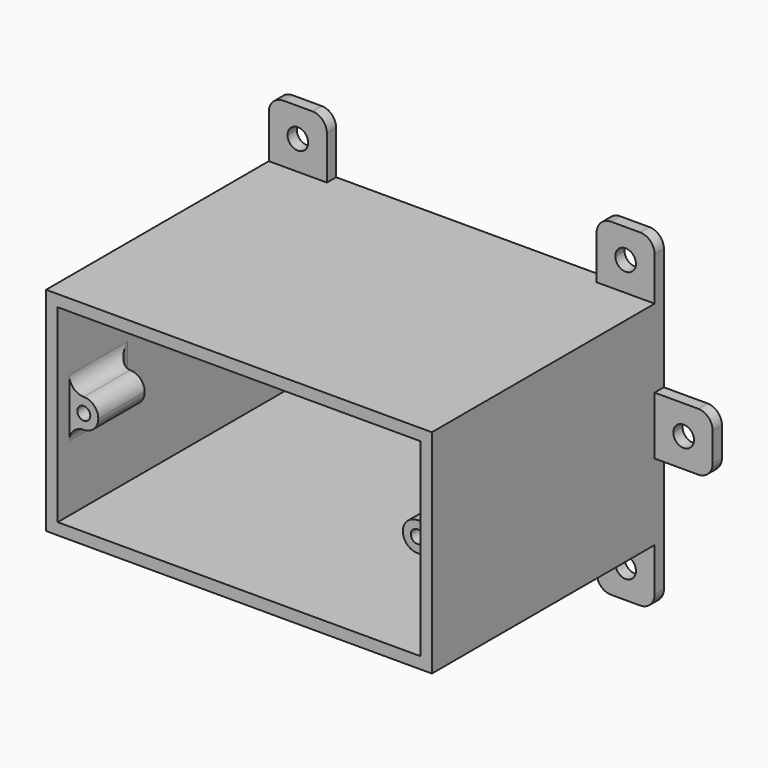
from build123d import *

# Parameters (mm, degrees)
F1_DEPTH     = 40
F0_W         = 8
F0_H         = 8
F0_R         = 1.425
F2_DEPTH     = 1.6
F3_R         = 2
F5_R         = 2
F6_START     = 30
F0_W_2       = 4
F0_H_2       = 4
F0_R_2       = 0.9
F6_DEPTH     = 8
F7_T1_DEPTH  = 8
F7_T6_DEPTH  = 4
F7_S7_R      = 0.9
F7_T8_DEPTH  = 4
F7_T13_DEPTH = 9
F7_T17_DEPTH = 13
F7_T24_DEPTH = 9
F7_T28_DEPTH = 13
F7_T31_DEPTH = 18


# Not quite as in the source:
# - a fillet or chamfer that OpenCascade refuses, or shapes differently, is made with other operations: its cross-section is extruded or revolved along the edge and cut away or added


with BuildPart() as f1:
    # F0 (on Front) → F1 (new body)
    with BuildSketch(Plane.XZ):
        Polygon((-26.6, -4.1515841149), (-26.6, -14.65), (-18.6, -14.65), (18.6, -14.65), (26.6, -14.65), (26.6, -4.1515841149), (26.6, 3.8484158851), (26.6, 14.65), (18.6, 14.65), (-18.6, 14.65), (-26.6, 14.65), (-26.6, 3.8484158851), align=None)
        Polygon((25, -2), (25, -13.05), (-25, -13.05), (-25, 13.05), (25, 13.05), (25, 2), align=None, mode=Mode.SUBTRACT)
    extrude(amount=F1_DEPTH)

    # F0 (on Front) → F2 (join)
    with BuildSketch(Plane.XZ):
        Polygon((-26.6, -4.1515841149), (-26.6, -14.65), (-18.6, -14.65), (18.6, -14.65), (26.6, -14.65), (26.6, -4.1515841149), (26.6, 3.8484158851), (26.6, 14.65), (18.6, 14.65), (-18.6, 14.65), (-26.6, 14.65), (-26.6, 3.8484158851), align=None)
        Polygon((25, -2), (25, -13.05), (-25, -13.05), (-25, 13.05), (25, 13.05), (25, 2), align=None, mode=Mode.SUBTRACT)
        with Locations((-22.6, -18.65)):
            Rectangle(F0_W, F0_H)
        with Locations((-22.6, -18.65)):
            Circle(F0_R, mode=Mode.SUBTRACT)
        with Locations((-30.6, -0.1515841149)):
            Rectangle(F0_W, F0_H)
        with Locations((-30.6, -0.1515841149)):
            Circle(F0_R, mode=Mode.SUBTRACT)
        with Locations((22.6, -18.65)):
            Rectangle(F0_W, F0_H)
        with Locations((22.6, -18.65)):
            Circle(F0_R, mode=Mode.SUBTRACT)
        with Locations((-22.6, 18.65)):
            Rectangle(F0_W, F0_H)
        with Locations((-22.6, 18.65)):
            Circle(F0_R, mode=Mode.SUBTRACT)
        with Locations((30.6, -0.1515841149)):
            Rectangle(F0_W, F0_H)
        with Locations((30.6, -0.1515841149)):
            Circle(F0_R, mode=Mode.SUBTRACT)
        with Locations((22.6, 18.65)):
            Rectangle(F0_W, F0_H)
        with Locations((22.6, 18.65)):
            Circle(F0_R, mode=Mode.SUBTRACT)
    extrude(amount=F2_DEPTH)

    # F3
    f3_edges = [f1.edges().sort_by_distance(p)[0] for p in [
        (-26.6, -0.8, 22.65),
        (-18.6, -0.8, 22.65),
        (18.6, -0.8, 22.65),
        (26.6, -0.8, 22.65),
        (34.6, -0.8, 3.848416),
        (34.6, -0.8, -4.151584),
        (26.6, -0.8, -22.65),
        (18.6, -0.8, -22.65),
        (-34.6, -0.8, -4.151584),
        (-34.6, -0.8, 3.848416),
        (-26.6, -0.8, -22.65),
    ]]
    fillet(f3_edges, radius=F3_R)

    # F4: F1 across plane


with BuildPart() as f1_1:
    add(f1.part)
    add(f1.part.mirror(Plane.YZ))

    # F5
    f5_edges = [f1_1.edges().sort_by_distance(p)[0] for p in [
        (-18.6, -0.8, -22.65),
        (18.6, -0.8, -22.65),
    ]]
    fillet(f5_edges, radius=F5_R)

    # F0 (on Front) → F6 (join)
    with BuildSketch(Plane.XZ.offset(F6_START)):
        with Locations((23, 0)):
            Rectangle(F0_W_2, F0_H_2)
        with Locations((23, 0)):
            Circle(F0_R_2, mode=Mode.SUBTRACT)
    extrude(amount=F6_DEPTH)

    # F7: fillet of radius 2 on 5 edges, made by hand

    # F7_s2 → F7_t1 (join)
    with BuildSketch(Plane.XZ.offset(30)):
        with BuildLine():
            ThreePointArc((25, -4), (24.4142135624, -2.5857864376), (23, -2))
            Line((23, -2), (25, -2))
            Line((25, -2), (25, -4))
        make_face()
        with BuildLine():
            ThreePointArc((25, 4), (24.4142135624, 2.5857864376), (23, 2))
            Line((23, 2), (25, 2))
            Line((25, 2), (25, 4))
        make_face()
    extrude(amount=F7_T1_DEPTH)


with BuildPart() as f7_tool4:
    # F7_s5 → F7_t6 (new body)
    with BuildSketch(Plane.XY.offset(-2)):
        with BuildLine():
            ThreePointArc((25, -28), (24.4142135624, -29.4142135624), (23, -30))
            Line((23, -30), (25, -30))
            Line((25, -30), (25, -28))
        make_face()
    extrude(amount=F7_T6_DEPTH)

    # F7_s7 → F7_t8 (cut, symmetric)
    with BuildSketch(Plane.XZ.offset(29)):
        with Locations((23, 0)):
            Circle(F7_S7_R)
    extrude(amount=F7_T8_DEPTH, both=True, mode=Mode.SUBTRACT)


with BuildPart() as f1_2:
    add(f1_1.part)

    # F7_t3: union F7_tool4
    add(f7_tool4.part)


with BuildPart() as f7_tool11:
    # F7_s12 → F7_t13 (new body)
    with BuildSketch(Plane.XY.offset(-7)):
        with BuildLine():
            ThreePointArc((25, -28), (24.4142135624, -29.4142135624), (23, -30))
            Line((23, -30), (25, -30))
            Line((25, -30), (25, -28))
        make_face()
    extrude(amount=F7_T13_DEPTH)

    split(bisect_by=Plane.XY.offset(-2), keep=Keep.BOTTOM)


with BuildPart() as f7_tool15:
    # F7_s16 → F7_t17 (new body)
    with BuildSketch(Plane.XZ.offset(25)):
        with BuildLine():
            ThreePointArc((25, -4), (24.4142135624, -2.5857864376), (23, -2))
            Line((23, -2), (25, -2))
            Line((25, -2), (25, -4))
        make_face()
    extrude(amount=F7_T17_DEPTH)

    split(bisect_by=Plane.XZ.offset(30), keep=Keep.BOTTOM)


with BuildPart() as f7_tool11_1:
    add(f7_tool11.part)

    # F7_t19: intersect F7_tool15
    add(f7_tool15.part, mode=Mode.INTERSECT)


with BuildPart() as f1_3:
    add(f1_2.part)

    # F7_t9: union F7_tool11
    add(f7_tool11_1.part)


with BuildPart() as f7_tool22:
    # F7_s23 → F7_t24 (new body)
    with BuildSketch(Plane.XY.offset(-2)):
        with BuildLine():
            ThreePointArc((25, -28), (24.4142135624, -29.4142135624), (23, -30))
            Line((23, -30), (25, -30))
            Line((25, -30), (25, -28))
        make_face()
    extrude(amount=F7_T24_DEPTH)

    split(bisect_by=Plane.XY.offset(2), keep=Keep.TOP)


with BuildPart() as f7_tool26:
    # F7_s27 → F7_t28 (new body)
    with BuildSketch(Plane.XZ.offset(25)):
        with BuildLine():
            ThreePointArc((25, 4), (24.4142135624, 2.5857864376), (23, 2))
            Line((23, 2), (25, 2))
            Line((25, 2), (25, 4))
        make_face()
    extrude(amount=F7_T28_DEPTH)

    split(bisect_by=Plane.XZ.offset(30), keep=Keep.BOTTOM)


with BuildPart() as f7_tool22_1:
    add(f7_tool22.part)

    # F7_t30: intersect F7_tool26
    add(f7_tool26.part, mode=Mode.INTERSECT)


with BuildPart() as f1_4:
    add(f1_3.part)

    # F7_t20: union F7_tool22
    add(f7_tool22_1.part)

    # F7_s32 → F7_t31 (cut)
    with BuildSketch(Plane.XZ.offset(25)):
        with BuildLine():
            ThreePointArc((23, -2), (21.5857864376, -1.4142135624), (21, 0))
            Line((21, 0), (21, -2))
            Line((21, -2), (23, -2))
        make_face()
        with BuildLine():
            ThreePointArc((23, 2), (21.5857864376, 1.4142135624), (21, 0))
            Line((21, 0), (21, 2))
            Line((21, 2), (23, 2))
        make_face()
    extrude(amount=F7_T31_DEPTH, mode=Mode.SUBTRACT)

    # F8: F1 across plane


with BuildPart() as f1_5:
    add(f1_4.part)
    add(f1_4.part.mirror(Plane.YZ))


solid = f1_5.part
